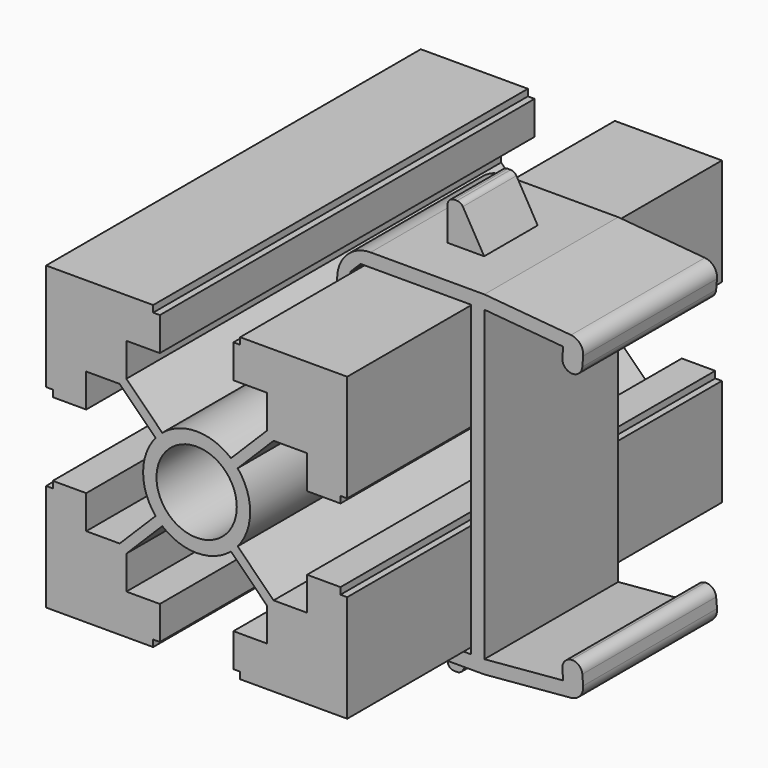
from build123d import *

# Parameters (mm, degrees)
F0_R         = 6
F1_DEPTH     = 35
F3_DEPTH     = 12.5
F4_DEPTH     = 5
F5_R         = 5
F6_R         = 0.5
F7_R         = 1
F8_R         = 1
F9_R         = 1.49999
F10_T1_DEPTH = 35


# Not quite as in the source:
# - a fillet or chamfer that OpenCascade refuses, or shapes differently, is made with other operations: its cross-section is extruded or revolved along the edge and cut away or added
# - a fillet or chamfer is up to 0.001 mm smaller than in the source, because OpenCascade refuses the exact size


with BuildPart() as f1:
    # F0 (on Front) → F1 (new body, symmetric)
    with BuildSketch(Plane.XZ):
        with BuildLine():
            Line((-6.5, 21.5), (-6.5, 22.5))
            Line((-6.5, 22.5), (-22.5, 22.5))
            Line((-22.5, 22.5), (-22.5, 6.5))
            Line((-22.5, 6.5), (-21.5, 6.5))
            Line((-21.5, 6.5), (-21.5, 5.5))
            Line((-21.5, 5.5), (-16.5, 5.5))
            Line((-16.5, 5.5), (-16.5, 10.5))
            Line((-16.5, 10.5), (-11.5, 10.5))
            Line((-11.5, 10.5), (-6.1347138348, 5.1347138348))
            ThreePointArc((-6.1347138348, 5.1347138348), (-5.6568542495, 5.6568542495), (-5.1347138348, 6.1347138348))
            Line((-5.1347138348, 6.1347138348), (-10.5, 11.5))
            Line((-10.5, 11.5), (-10.5, 16.5))
            Line((-10.5, 16.5), (-5.5, 16.5))
            Line((-5.5, 16.5), (-5.5, 21.5))
            Line((-5.5, 21.5), (-6.5, 21.5))
        make_face()
        with BuildLine():
            ThreePointArc((5.1347138348, 6.1347138348), (0, 8), (-5.1347138348, 6.1347138348))
            ThreePointArc((-5.1347138348, 6.1347138348), (-5.6568542495, 5.6568542495), (-6.1347138348, 5.1347138348))
            ThreePointArc((-6.1347138348, 5.1347138348), (-8, 0), (-6.1347138348, -5.1347138348))
            ThreePointArc((-6.1347138348, -5.1347138348), (-5.6568542495, -5.6568542495), (-5.1347138348, -6.1347138348))
            ThreePointArc((-5.1347138348, -6.1347138348), (0, -8), (5.1347138348, -6.1347138348))
            ThreePointArc((5.1347138348, -6.1347138348), (5.6568542495, -5.6568542495), (6.1347138348, -5.1347138348))
            ThreePointArc((6.1347138348, -5.1347138348), (7.5192323637, -2.7315095938), (8, 0))
            ThreePointArc((8, 0), (7.5192323637, 2.7315095938), (6.1347138348, 5.1347138348))
            ThreePointArc((6.1347138348, 5.1347138348), (5.6568542495, 5.6568542495), (5.1347138348, 6.1347138348))
        make_face()
        Circle(F0_R, mode=Mode.SUBTRACT)
        with BuildLine():
            Line((10.5, 11.5), (5.1347138348, 6.1347138348))
            ThreePointArc((5.1347138348, 6.1347138348), (5.6568542495, 5.6568542495), (6.1347138348, 5.1347138348))
            Line((6.1347138348, 5.1347138348), (11.5, 10.5))
            Line((11.5, 10.5), (16.5, 10.5))
            Line((16.5, 10.5), (16.5, 5.5))
            Line((16.5, 5.5), (21.5, 5.5))
            Line((21.5, 5.5), (21.5, 6.5))
            Line((21.5, 6.5), (22.5, 6.5))
            Line((22.5, 6.5), (22.5, 22.5))
            Line((22.5, 22.5), (6.5, 22.5))
            Line((6.5, 22.5), (6.5, 21.5))
            Line((6.5, 21.5), (5.5, 21.5))
            Line((5.5, 21.5), (5.5, 16.5))
            Line((5.5, 16.5), (10.5, 16.5))
            Line((10.5, 16.5), (10.5, 11.5))
        make_face()
        with BuildLine():
            ThreePointArc((-5.1347138348, -6.1347138348), (-5.6568542495, -5.6568542495), (-6.1347138348, -5.1347138348))
            Line((-6.1347138348, -5.1347138348), (-11.5, -10.5))
            Line((-11.5, -10.5), (-16.5, -10.5))
            Line((-16.5, -10.5), (-16.5, -5.5))
            Line((-16.5, -5.5), (-21.5, -5.5))
            Line((-21.5, -5.5), (-21.5, -6.5))
            Line((-21.5, -6.5), (-22.5, -6.5))
            Line((-22.5, -6.5), (-22.5, -22.5))
            Line((-22.5, -22.5), (-6.5, -22.5))
            Line((-6.5, -22.5), (-6.5, -21.5))
            Line((-6.5, -21.5), (-5.5, -21.5))
            Line((-5.5, -21.5), (-5.5, -16.5))
            Line((-5.5, -16.5), (-10.5, -16.5))
            Line((-10.5, -16.5), (-10.5, -11.5))
            Line((-10.5, -11.5), (-5.1347138348, -6.1347138348))
        make_face()
        with BuildLine():
            Line((11.5, -10.5), (6.1347138348, -5.1347138348))
            ThreePointArc((6.1347138348, -5.1347138348), (5.6568542495, -5.6568542495), (5.1347138348, -6.1347138348))
            Line((5.1347138348, -6.1347138348), (10.5, -11.5))
            Line((10.5, -11.5), (10.5, -16.5))
            Line((10.5, -16.5), (5.5, -16.5))
            Line((5.5, -16.5), (5.5, -21.5))
            Line((5.5, -21.5), (6.5, -21.5))
            Line((6.5, -21.5), (6.5, -22.5))
            Line((6.5, -22.5), (22.5, -22.5))
            Line((22.5, -22.5), (22.5, -6.5))
            Line((22.5, -6.5), (21.5, -6.5))
            Line((21.5, -6.5), (21.5, -5.5))
            Line((21.5, -5.5), (16.5, -5.5))
            Line((16.5, -5.5), (16.5, -10.5))
            Line((16.5, -10.5), (11.5, -10.5))
        make_face()
    extrude(amount=F1_DEPTH, both=True)


with BuildPart() as f3:
    # F2 (on Front) → F3 (new body, symmetric)
    with BuildSketch(Plane.XZ):
        Polygon((5, 16), (5, 21.5), (6.5, 23), (23, 23), (23, 0), (23, -23), (6.5, -23), (5, -21.5), (5, -16), (10, -16), (3, -9.5), (3, -21.5), (3, -25), (6.5, -25), (13.5, -25), (18.9641016151, -25), (22.5, -25), (25, -25), (25, -22.9923603249), (25, -22.5), (25, 0), (25, 22.5), (25, 22.9923603249), (25, 25), (22.5, 25), (18.9641016151, 25), (15.5, 25), (14.5, 25), (13.5, 25), (6.5, 25), (3, 25), (3, 21.5), (3, 9.5), (10, 16), align=None)
        Polygon((39.9429204714, 23.6926638588), (25, 25), (25, 22.9923603249), (36.7800248916, 21.9617416908), (39.7686089859, 21.7002744626), align=None)
        Polygon((39.7686089859, 21.7002744626), (36.7800248916, 21.9617416908), (36.5185576634, 18.9731575966), (39.5071417576, 18.7116903683), align=None)
        Polygon((25, -22.9923603249), (25, -25), (39.9429204714, -23.6926638588), (39.7686089859, -21.7002744626), (36.7800248916, -21.9617416908), align=None)
        Polygon((36.5185576634, -18.9731575966), (36.7800248916, -21.9617416908), (39.7686089859, -21.7002744626), (39.5071417576, -18.7116903683), align=None)
    extrude(amount=F3_DEPTH, both=True)

    # F2 (on Front) → F4 (join, symmetric)
    with BuildSketch(Plane.XZ):
        Polygon((13.5, 31), (13.5, 25), (14.5, 25), (15.5, 25), (18.9641016151, 25), (15.5, 31), align=None)
        Polygon((18.9641016151, -25), (13.5, -25), (13.5, -31), (15.5, -31), align=None)
    extrude(amount=F4_DEPTH, both=True)

    # F5
    f5_edges = [f3.edges().sort_by_distance(p)[0] for p in [
        (3, 0, 25),
        (3, 0, -25),
    ]]
    fillet(f5_edges, radius=F5_R)

    # F6
    f6_edges = [f3.edges().sort_by_distance(p)[0] for p in [
        (10, 0, 16),
        (10, 0, -16),
    ]]
    fillet(f6_edges, radius=F6_R)

    # F7
    f7_edges = [f3.edges().sort_by_distance(p)[0] for p in [
        (3, 0, 9.5),
        (3, 0, -9.5),
    ]]
    fillet(f7_edges, radius=F7_R)

    # F8
    f8_edges = [f3.edges().sort_by_distance(p)[0] for p in [
        (13.5, 0, 31),
        (15.5, 0, 31),
        (15.5, 0, -31),
        (13.5, 0, -31),
    ]]
    fillet(f8_edges, radius=F8_R)

    # F9 (radius 1.5 in the source; OpenCascade refuses exactly that, so slightly less here)
    f9_edges = [f3.edges().sort_by_distance(p)[0] for p in [
        (39.507142, 0, 18.71169),
        (36.518558, 0, 18.973158),
        (39.507142, 0, -18.71169),
        (36.518558, 0, -18.973158),
    ]]
    fillet(f9_edges, radius=F9_R)

    # F10: fillet of radius 2 on 2 edges, made by hand

    # F10_s2 → F10_t1 (cut)
    with BuildSketch(Plane.XZ.offset(-17.5)):
        with BuildLine():
            ThreePointArc((39.7686089859, 21.7002744626), (39.3083084759, 23.1601611675), (37.9505310752, 23.8669753443))
            Line((37.9505310752, 23.8669753443), (39.9429204714, 23.6926638588))
            Line((39.9429204714, 23.6926638588), (39.7686089859, 21.7002744626))
        make_face()
        with BuildLine():
            ThreePointArc((39.7686089859, -21.7002744626), (39.3083084759, -23.1601611675), (37.9505310752, -23.8669753443))
            Line((37.9505310752, -23.8669753443), (39.9429204714, -23.6926638588))
            Line((39.9429204714, -23.6926638588), (39.7686089859, -21.7002744626))
        make_face()
    extrude(amount=F10_T1_DEPTH, mode=Mode.SUBTRACT)


solid = Compound([f1.part, f3.part])
